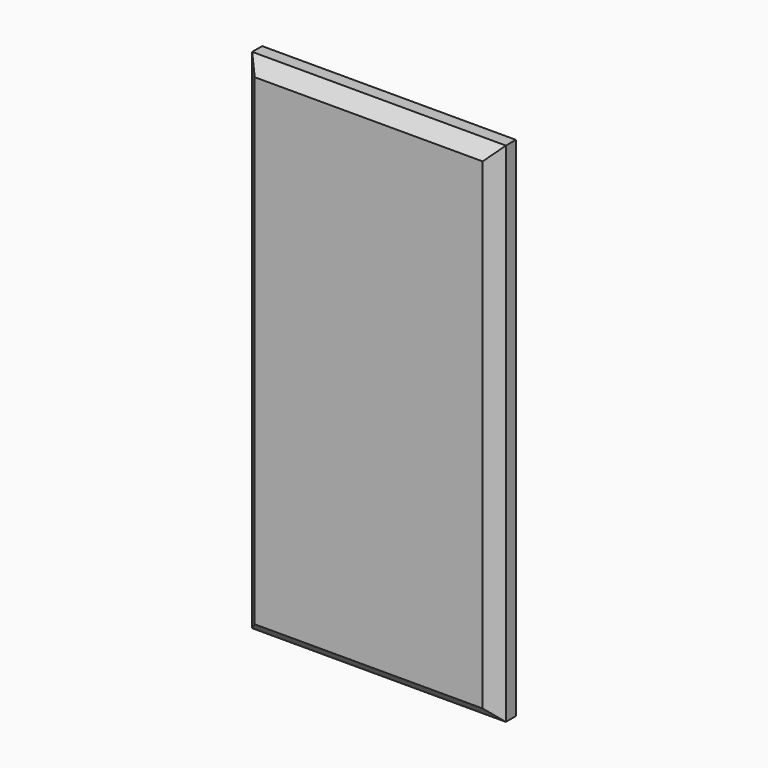
from build123d import *

# Parameters (mm, degrees)
F0_W     = 100
F0_H     = 200
F1_DEPTH = 10
F2_SIZE  = 5.08


# Not quite as in the source:
# - the program builds the solid bodies; features that only make, move or delete a surface that nothing else refers to are left out


with BuildPart() as f1:
    # F0 (on Front) → F1 (new body)
    with BuildSketch(Plane.XZ):
        Rectangle(F0_W, F0_H)
    extrude(amount=F1_DEPTH)

    # F2
    f2_edges = [f1.edges().sort_by_distance(p)[0] for p in [
        (-50, -10, 0),
        (0, -10, 100),
        (0, -10, -100),
        (50, -10, 0),
    ]]
    chamfer(f2_edges, length=F2_SIZE)


solid = f1.part
